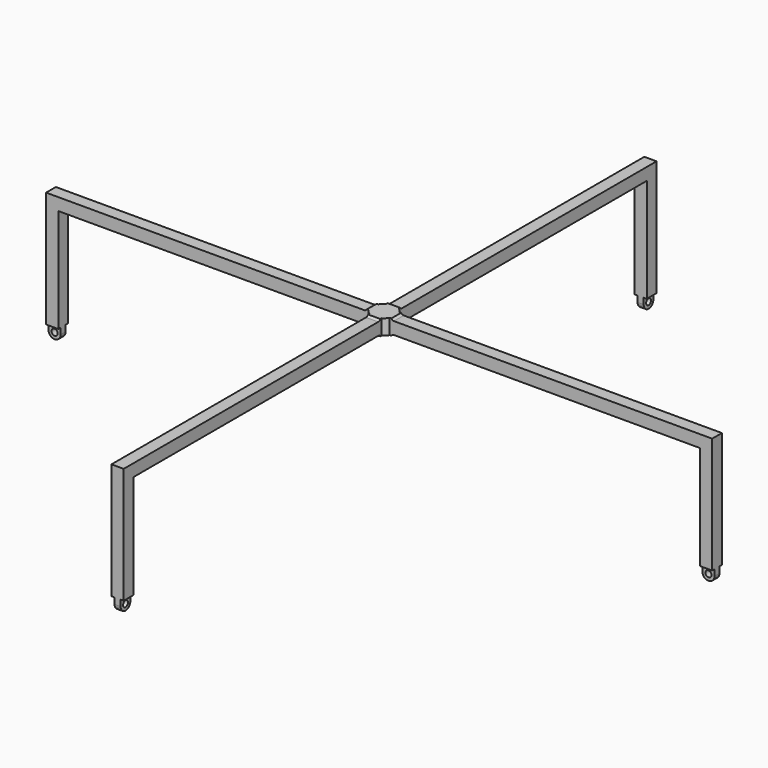
from build123d import *

# Parameters (mm, degrees)
F0_R            = 5
F1_DEPTH        = 20
F2_T1_DEPTH     = 20
F4_COUNT        = 4
F3_R            = 20
F5_DEPTH        = 25
F6_R            = 5
F7_DEPTH        = 5
F7_COPIES_COUNT = 4
F8_W            = 20
F8_H            = 20
F9_DEPTH        = 5
F9_COPIES_COUNT = 4


# Not quite as in the source:
# - a fillet or chamfer that OpenCascade refuses, or shapes differently, is made with other operations: its cross-section is extruded or revolved along the edge and cut away or added
# - a pattern or mirror of a feature is missing from the dataset's text; its kind, count and spacing are read off the source's solid


with BuildPart() as f1:
    # F0 (on Front) → F1 (new body)
    with BuildSketch(Plane.XZ):
        with BuildLine():
            Line((0, 25), (0, 0))
            Line((0, 0), (20, 0))
            Line((20, 0), (20, 2.5))
            Line((20, 2.5), (525, 2.5))
            Line((525, 2.5), (525, -177.5))
            ThreePointArc((525, -177.5), (535, -187.5), (545, -177.5))
            Line((545, -177.5), (545, 22.5))
            Line((545, 22.5), (20, 22.5))
            Line((20, 22.5), (20, 25))
            Line((20, 25), (0, 25))
        make_face()
        with Locations((535, -177.5)):
            Circle(F0_R, mode=Mode.SUBTRACT)
    extrude(amount=F1_DEPTH)

    # F2: fillet of radius 5 on 2 edges, made by hand

    # F2_s2 → F2_t1 (join)
    with BuildSketch(Plane.XZ):
        with BuildLine():
            ThreePointArc((24.3301270189, 22.5), (21.8301270189, 23.1698729811), (20, 25))
            Line((20, 25), (20, 22.5))
            Line((20, 22.5), (24.3301270189, 22.5))
        make_face()
        with BuildLine():
            ThreePointArc((20, 0), (21.8301270189, 1.8301270189), (24.3301270189, 2.5))
            Line((24.3301270189, 2.5), (20, 2.5))
            Line((20, 2.5), (20, 0))
        make_face()
    extrude(amount=F2_T1_DEPTH)

    # F4: F1 ×4 about axis
    f4_axis = Axis((0, -10, 25), (0, 0, 1))


with BuildPart() as f1_1:
    add(f1.part)
    for i in range(1, F4_COUNT):
        add(f1.part.rotate(f4_axis, i * 360 / F4_COUNT))

    # F3 (on face) → F5 (join, through all)
    with BuildSketch(Plane.XY.offset(25)):
        with Locations((0, -10)):
            Circle(F3_R)
    extrude(amount=-F5_DEPTH)

    # F6 (on face) → F7 (cut)
    with BuildSketch(Plane(origin=(-10, 0, 0), x_dir=(0, -1, 0), z_dir=(-1, 0, 0))):
        with BuildLine():
            Line((555, -177.5), (555, -167.5))
            Line((555, -167.5), (535, -167.5))
            Line((535, -167.5), (535, -177.5))
            ThreePointArc((535, -177.5), (537.9289321881, -184.5710678119), (545, -187.5))
            ThreePointArc((545, -187.5), (552.0710678119, -184.5710678119), (555, -177.5))
        make_face()
        with Locations((545, -177.5)):
            Circle(F6_R, mode=Mode.SUBTRACT)
    f7 = extrude(amount=-F7_DEPTH, mode=Mode.SUBTRACT)

    # F7_copies: F7 ×4 about axis
    f7_copies_axis = Axis((0, -10, 0), (0, 0, 1))
    for i in range(1, F7_COPIES_COUNT):
        add(f7.rotate(f7_copies_axis, i * 360 / F7_COPIES_COUNT), mode=Mode.SUBTRACT)

    # F8 (on face) → F9 (cut)
    with BuildSketch(Plane.YZ.offset(10)):
        with Locations((-545, -177.5)):
            Rectangle(F8_W, F8_H)
    f9 = extrude(amount=-F9_DEPTH, mode=Mode.SUBTRACT)

    # F9_copies: F9 ×4 about axis
    f9_copies_axis = Axis((0, -10, 0), (0, 0, 1))
    for i in range(1, F9_COPIES_COUNT):
        add(f9.rotate(f9_copies_axis, i * 360 / F9_COPIES_COUNT), mode=Mode.SUBTRACT)


solid = f1_1.part
